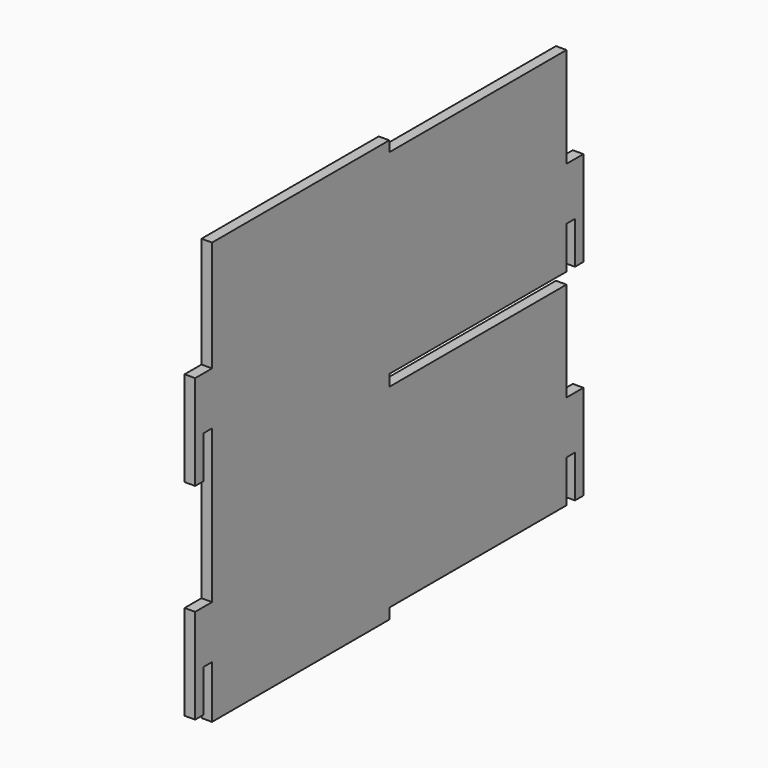
from build123d import *

# Parameters (mm, degrees)
F0_W     = 133.35
F0_H     = 6.35
F0_H_2   = 60.325
F0_H_3   = 31.75
F0_W_2   = 6.35
F0_H_4   = 25.4
F0_H_5   = 6.8349212326
F0_H_6   = 59.8400787674
F1_DEPTH = 6.35


# Not quite as in the source:
# - a feature names something its author has since deleted; it is built from what else it names


with BuildPart() as f1:
    # F0 (on Right) → F1 (new body)
    with BuildSketch(Plane.YZ):
        with Locations((-66.675, 123.825)):
            Rectangle(F0_W, F0_H)
        with Locations((-66.675, 90.4875)):
            Rectangle(F0_W, F0_H_2)
        with Locations((66.675, 90.4875)):
            Rectangle(F0_W, F0_H_2)
        with Locations((-66.675, 44.45)):
            Rectangle(F0_W, F0_H_3)
        with Locations((-136.525, 44.45)):
            Rectangle(F0_W_2, F0_H_3)
        with Locations((66.675, 44.45)):
            Rectangle(F0_W, F0_H_3)
        with Locations((-66.675, 15.875)):
            Rectangle(F0_W, F0_H_4)
        with Locations((-142.875, 44.45)):
            Rectangle(F0_W_2, F0_H_3)
        with Locations((136.525, 44.45)):
            Rectangle(F0_W_2, F0_H_3)
        with Locations((66.675, 15.875)):
            Rectangle(F0_W, F0_H_4)
        with Locations((-66.675, -0.2424606163)):
            Rectangle(F0_W, F0_H_5)
        with Locations((-142.875, 15.875)):
            Rectangle(F0_W_2, F0_H_4)
        Polygon((146.05, 60.325), (139.7, 60.325), (139.7, 28.575), (139.7, 3.175), (146.05, 3.175), align=None)
        with Locations((-66.675, -33.5799606163)):
            Rectangle(F0_W, F0_H_6)
        with Locations((66.675, -33.5799606163)):
            Rectangle(F0_W, F0_H_6)
        with Locations((-66.675, -79.375)):
            Rectangle(F0_W, F0_H_3)
        with Locations((-136.525, -79.375)):
            Rectangle(F0_W_2, F0_H_3)
        with Locations((66.675, -79.375)):
            Rectangle(F0_W, F0_H_3)
        with Locations((-66.675, -107.95)):
            Rectangle(F0_W, F0_H_4)
        with Locations((-142.875, -79.375)):
            Rectangle(F0_W_2, F0_H_3)
        with Locations((136.525, -79.375)):
            Rectangle(F0_W_2, F0_H_3)
        with Locations((66.675, -107.95)):
            Rectangle(F0_W, F0_H_4)
        with Locations((-66.675, -123.825)):
            Rectangle(F0_W, F0_H)
        with Locations((-142.875, -107.95)):
            Rectangle(F0_W_2, F0_H_4)
        Polygon((146.05, -63.5), (139.7, -63.5), (139.7, -95.25), (139.7, -120.65), (146.05, -120.65), align=None)
    extrude(amount=F1_DEPTH)


solid = f1.part
